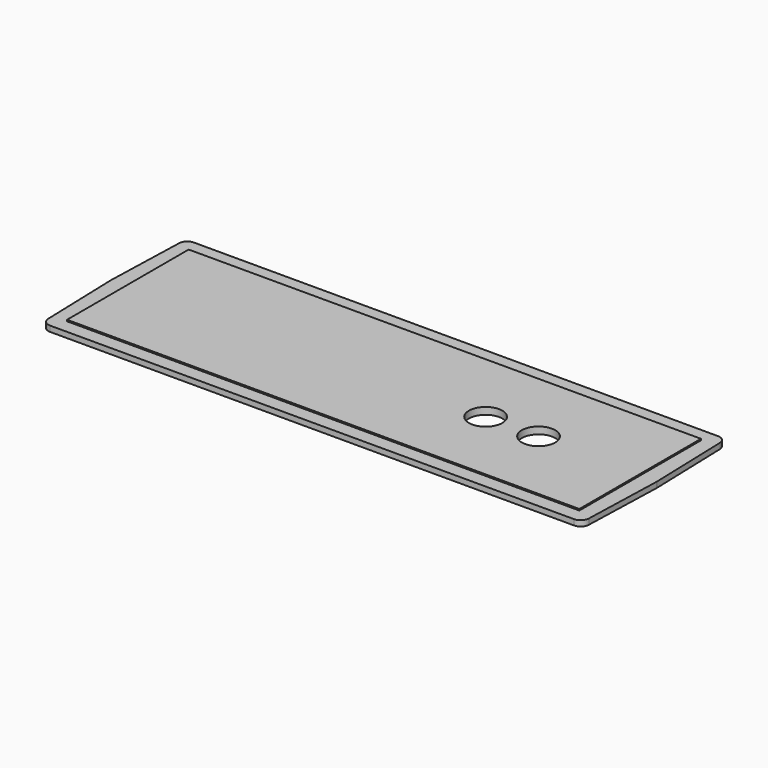
from build123d import *

# Parameters (mm, degrees)
F0_W        = 194
F0_H        = 64.6
F1_DEPTH    = 2
F2_W        = 184
F2_H        = 54.6
F3_DEPTH    = 0.5
F4_R        = 6
F5_DEPTH    = 25
F6_T1_DEPTH = 16.5427907903
F6_T3_DEPTH = 2.4643962848


# Not quite as in the source:
# - a fillet or chamfer that OpenCascade refuses, or shapes differently, is made with other operations: its cross-section is extruded or revolved along the edge and cut away or added


with BuildPart() as f1:
    # F0 (on Top) → F1 (new body)
    with BuildSketch(Plane.XY):
        Rectangle(F0_W, F0_H)
        Polygon((98, 0), (97, 32.3), (97, -32.3), align=None)
        Polygon((-97, -32.3), (-97, 32.3), (-98, 0), align=None)
    extrude(amount=F1_DEPTH)

    # F2 (on face) → F3 (join)
    with BuildSketch(Plane.XY.offset(2)):
        Rectangle(F2_W, F2_H)
    extrude(amount=F3_DEPTH)

    # F4 (on face) → F5 (cut)
    with BuildSketch(Plane.XY.offset(2.5)):
        with Locations((36.5, 0)):
            Circle(F4_R)
        with Locations((55.5, 0)):
            Circle(F4_R)
    extrude(amount=-F5_DEPTH, mode=Mode.SUBTRACT)

    # F6: fillet of radius 3 on 6 edges, made by hand

    # F6_s2 → F6_t1 (cut)
    with BuildSketch(Plane.XY.offset(-7.2713953952)):
        with BuildLine():
            ThreePointArc((97.0900051153, -29.3928347763), (96.1796822102, -31.4538923289), (94.0914418419, -32.3))
            Line((94.0914418419, -32.3), (97, -32.3))
            Line((97, -32.3), (97.0900051153, -29.3928347763))
        make_face()
        with BuildLine():
            ThreePointArc((94.0914418419, 32.3), (96.1796822102, 31.4538923289), (97.0900051153, 29.3928347763))
            Line((97.0900051153, 29.3928347763), (97, 32.3))
            Line((97, 32.3), (94.0914418419, 32.3))
        make_face()
        with BuildLine():
            ThreePointArc((-94.0914418419, 32.3), (-96.1796822102, 31.4538923289), (-97.0900051153, 29.3928347763))
            Line((-97.0900051153, 29.3928347763), (-97, 32.3))
            Line((-97, 32.3), (-94.0914418419, 32.3))
        make_face()
        with BuildLine():
            ThreePointArc((-97.0900051153, -29.3928347763), (-96.1796822102, -31.4538923289), (-94.0914418419, -32.3))
            Line((-94.0914418419, -32.3), (-97, -32.3))
            Line((-97, -32.3), (-97.0900051153, -29.3928347763))
        make_face()
    extrude(amount=F6_T1_DEPTH, mode=Mode.SUBTRACT)

    # F6_s4 → F6_t3 (cut)
    with BuildSketch(Plane.XY.offset(-0.2321981424)):
        with BuildLine():
            ThreePointArc((-97.9971258583, 0.0928347763), (-97.998562585, 0), (-97.9971258583, -0.0928347763))
            Line((-97.9971258583, -0.0928347763), (-98, 0))
            Line((-98, 0), (-97.9971258583, 0.0928347763))
        make_face()
        with BuildLine():
            ThreePointArc((97.9971258583, 0.0928347763), (97.998562585, 0), (97.9971258583, -0.0928347763))
            Line((97.9971258583, -0.0928347763), (98, 0))
            Line((98, 0), (97.9971258583, 0.0928347763))
        make_face()
    extrude(amount=F6_T3_DEPTH, mode=Mode.SUBTRACT)


solid = f1.part
